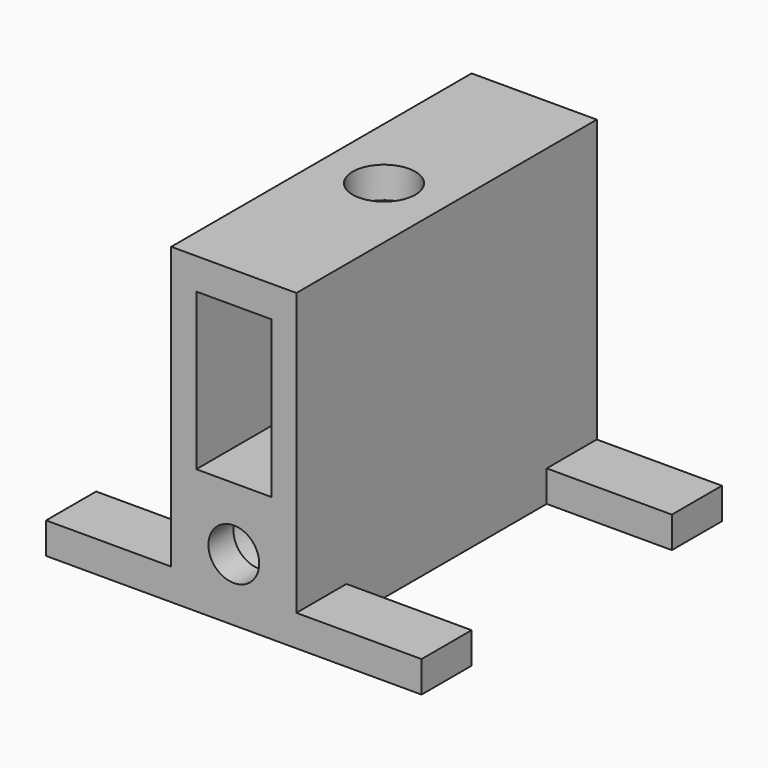
from build123d import *

# Parameters (mm, degrees)
F0_W           = 25.4
F0_H           = 76.2
F1_DEPTH       = 25.4
F2_W           = 25.4
F2_H           = 12.7
F3_DEPTH       = 6.35
F5_START       = -6.35
F4_R           = 9.525
F5_DEPTH       = 63.5
F6_R           = 5.1562
F7_DEPTH       = 76.201
F9_W           = 5.08
F9_H           = 76.2
F10_DEPTH      = 38.1
F11_W          = 20.32
F11_H          = 76.2
F12_DEPTH      = 6.35
F8_R           = 6.35
F13_DEPTH      = 5.6014842716
F13_DEPTH_BACK = 38.101


with BuildPart() as f1:
    # F0 (on Top) → F1 (new body)
    with BuildSketch(Plane.XY):
        with Locations((12.7, 38.1)):
            Rectangle(F0_W, F0_H)
    extrude(amount=F1_DEPTH)

    # F2 (on Top) → F3 (join)
    with BuildSketch(Plane.XY):
        with Locations((-12.7, 6.35)):
            Rectangle(F2_W, F2_H)
        with Locations((38.1, 6.35)):
            Rectangle(F2_W, F2_H)
        with Locations((-12.7, 69.85)):
            Rectangle(F2_W, F2_H)
        with Locations((38.1, 69.85)):
            Rectangle(F2_W, F2_H)
    extrude(amount=F3_DEPTH)

    # F4 (on face) → F5 (cut)
    with BuildSketch(Plane.XZ.offset(F5_START)):
        with Locations((12.7, 12.7)):
            Circle(F4_R)
    extrude(amount=-F5_DEPTH, mode=Mode.SUBTRACT)

    # F6 (on face) → F7 (cut, through all)
    with BuildSketch(Plane.XZ):
        with Locations((12.7, 12.7)):
            Circle(F6_R)
    extrude(amount=-F7_DEPTH, mode=Mode.SUBTRACT)

    # F9 (on face) → F10 (join)
    with BuildSketch(Plane.XY.offset(25.4)):
        with Locations((22.86, 38.1)):
            Rectangle(F9_W, F9_H)
        with Locations((2.54, 38.1)):
            Rectangle(F9_W, F9_H)
    extrude(amount=F10_DEPTH)

    # F11 (on face) → F12 (join)
    with BuildSketch(Plane.XY.offset(63.5)):
        with Locations((10.16, 38.1)):
            Rectangle(F11_W, F11_H)
    extrude(amount=-F12_DEPTH)

    # F8 (on face) → F13 (cut, two sides)
    with BuildSketch(Plane.XY.offset(25.4)) as f13_sk:
        with Locations((12.7, 38.1)):
            Circle(F8_R)
    extrude(amount=-F13_DEPTH, mode=Mode.SUBTRACT)
    extrude(f13_sk.sketch, amount=F13_DEPTH_BACK, mode=Mode.SUBTRACT)


solid = f1.part
